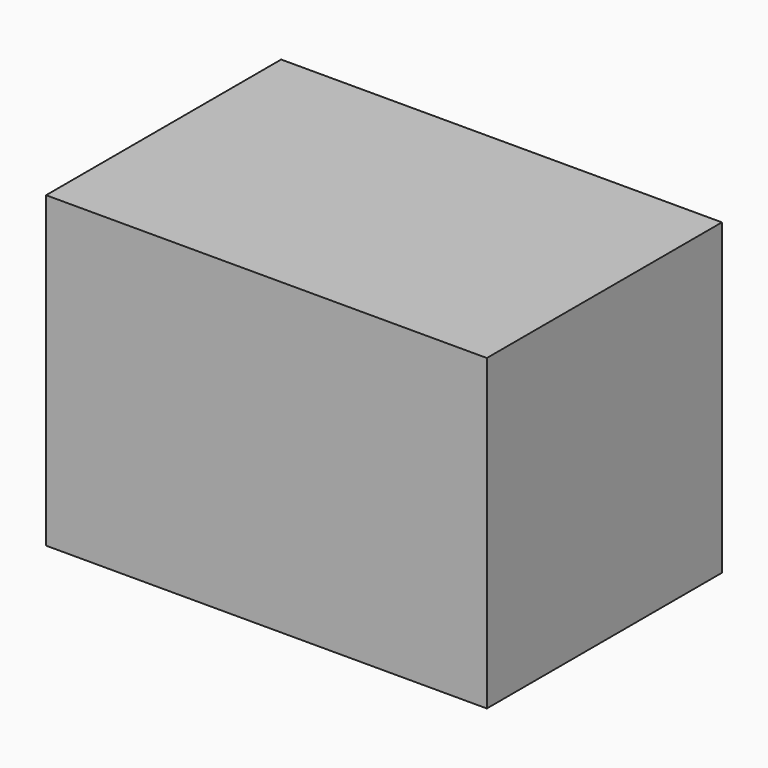
from build123d import *

# Parameters (mm, degrees)
F1_DEPTH = 30
F2_DEPTH = 1


# Not quite as in the source:
# - a feature names something its author has since deleted; it is built from what else it names


with BuildPart() as f1:
    # F0 (on Right) → F1 (new body)
    with BuildSketch(Plane.YZ):
        Polygon((10, 5), (0, 5), (-10, 5), (-10, -15), (10, -15), align=None)
    extrude(amount=F1_DEPTH)

    # F2 (add): a face of the model
    f2_faces = [f1.faces().sort_by_distance(p)[0] for p in [
        (15, 0, 5),
    ]]
    extrude(f2_faces, amount=F2_DEPTH)


solid = f1.part
